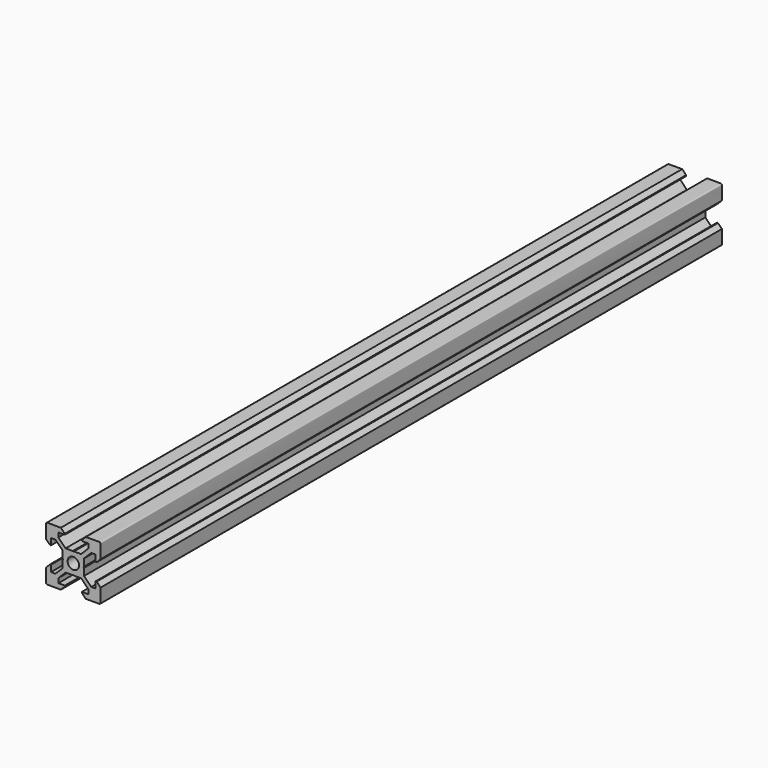
from build123d import *

# Parameters (mm, degrees)
F1_DEPTH = 284.8


# Not quite as in the source:
# - the dataset's text gives a spline's control points without its knots; the knots are read off the source's solid


with BuildPart() as f1:
    # F0 (on Front) → F1 (new body)
    with BuildSketch(Plane.XZ):
        with BuildLine():
            add(Edge.make_bspline(
                [(-8.545, 3.1250000004), (-8.43, 3.1250000004), (-8.315, 3.1250000004), (-8.2, 3.1250000004)],
                knots=[0, 0, 0, 0, 1, 1, 1, 1], degree=3))
            add(Edge.make_bspline(
                [(-8.2, 3.1250000004), (-8.2, 3.9166666671), (-8.2, 4.7083333338), (-8.2, 5.5000000004)],
                knots=[0, 0, 0, 0, 1, 1, 1, 1], degree=3))
            add(Edge.make_bspline(
                [(-8.1999999959, 5.5000000044), (-7.6535533893, 5.5000000044), (-7.1071067826, 5.5000000044), (-6.5606601759, 5.5000000044)],
                knots=[0, 0, 0, 0, 1, 1, 1, 1], degree=3))
            add(Edge.make_bspline(
                [(-6.5606601759, 5.5000000044), (-5.6737734493, 4.6131132778), (-4.7868867226, 3.7262265511), (-3.8999999959, 2.8393398244)],
                knots=[0, 0, 0, 0, 1, 1, 1, 1], degree=3))
            add(Edge.make_bspline(
                [(-3.8999999979, 2.8393398226), (-3.8999999979, 1.9628932159), (-3.8999999979, 1.0864466093), (-3.8999999979, 0.2100000026)],
                knots=[0, 0, 0, 0, 1, 1, 1, 1], degree=3))
            add(Edge.make_bspline(
                [(-3.9, 0.2100000008), (-3.83, 0.1400000008), (-3.76, 0.0700000008), (-3.69, 8e-10)],
                knots=[0, 0, 0, 0, 1, 1, 1, 1], degree=3))
            add(Edge.make_bspline(
                [(-3.9, -0.2099999992), (-3.83, -0.1399999992), (-3.76, -0.0699999992), (-3.69, 8e-10)],
                knots=[0, 0, 0, 0, 1, 1, 1, 1], degree=3))
            add(Edge.make_bspline(
                [(-3.8999999991, -2.839339821), (-3.8999999987, -1.9628932143), (-3.8999999984, -1.0864466077), (-3.899999998, -0.210000001)],
                knots=[0, 0, 0, 0, 1, 1, 1, 1], degree=3))
            add(Edge.make_bspline(
                [(-6.5606601782, -5.5000000017), (-5.6737734512, -4.6131132754), (-4.7868867241, -3.7262265491), (-3.8999999971, -2.8393398228)],
                knots=[0, 0, 0, 0, 1, 1, 1, 1], degree=3))
            add(Edge.make_bspline(
                [(-8.1999999982, -5.5000000011), (-7.6535533915, -5.5000000013), (-7.1071067849, -5.5000000015), (-6.5606601782, -5.5000000017)],
                knots=[0, 0, 0, 0, 1, 1, 1, 1], degree=3))
            add(Edge.make_bspline(
                [(-8.2000000012, -3.1249999971), (-8.2000000015, -3.9166666637), (-8.2000000019, -4.7083333304), (-8.2000000022, -5.4999999971)],
                knots=[0, 0, 0, 0, 1, 1, 1, 1], degree=3))
            add(Edge.make_bspline(
                [(-8.5450000012, -3.1249999969), (-8.4300000012, -3.124999997), (-8.3150000012, -3.124999997), (-8.2000000012, -3.1249999971)],
                knots=[0, 0, 0, 0, 1, 1, 1, 1], degree=3))
            add(Edge.make_bspline(
                [(-10.0000000018, -4.5799999963), (-9.5150000016, -4.0949999965), (-9.0300000014, -3.6099999967), (-8.5450000012, -3.1249999969)],
                knots=[0, 0, 0, 0, 1, 1, 1, 1], degree=3))
            add(Edge.make_bspline(
                [(-10.0000000038, -9.4999999963), (-10.0000000032, -7.8599999963), (-10.0000000025, -6.2199999963), (-10.0000000018, -4.5799999963)],
                knots=[0, 0, 0, 0, 1, 1, 1, 1], degree=3))
            add(Edge.make_bspline(
                [(-9.5000000039, -9.9999999965), (-9.5655199967, -9.9999999965), (-9.6293005688, -9.9873132519), (-9.6913417201, -9.9619397628), (-9.7513299005, -9.9374058943), (-9.8054004587, -9.9012771024), (-9.8535533945, -9.853553387), (-9.8995865416, -9.8079305653), (-9.9357153335, -9.7538600072), (-9.9619397702, -9.6913417126), (-9.9873132593, -9.6308520521), (-10.0000000039, -9.56707148), (-10.0000000038, -9.4999999963)],
                knots=[0, 0, 0, 0, 0.25, 0.25, 0.25, 0.5, 0.5, 0.5, 0.75, 0.75, 0.75, 1, 1, 1, 1], degree=3))
            add(Edge.make_bspline(
                [(-4.580000004, -9.9999999986), (-6.220000004, -9.9999999979), (-7.860000004, -9.9999999972), (-9.500000004, -9.9999999965)],
                knots=[0, 0, 0, 0, 1, 1, 1, 1], degree=3))
            Line((-4.580000004, -9.9999999986), (-3.1250000034, -8.5449999991))
            add(Edge.make_bspline(
                [(-3.1250000033, -8.1999999991), (-3.1250000033, -8.3149999991), (-3.1250000034, -8.4299999991), (-3.1250000034, -8.5449999991)],
                knots=[0, 0, 0, 0, 1, 1, 1, 1], degree=3))
            add(Edge.make_bspline(
                [(-5.5000000033, -8.1999999982), (-4.7083333366, -8.1999999985), (-3.91666667, -8.1999999988), (-3.1250000033, -8.1999999991)],
                knots=[0, 0, 0, 0, 1, 1, 1, 1], degree=3))
            add(Edge.make_bspline(
                [(-5.5000000066, -6.5606601742), (-5.5000000069, -7.1071067808), (-5.5000000071, -7.6535533875), (-5.5000000073, -8.1999999942)],
                knots=[0, 0, 0, 0, 1, 1, 1, 1], degree=3))
            add(Edge.make_bspline(
                [(-2.8393398255, -3.8999999953), (-3.7262265526, -4.7868867216), (-4.6131132796, -5.6737734479), (-5.5000000066, -6.5606601742)],
                knots=[0, 0, 0, 0, 1, 1, 1, 1], degree=3))
            add(Edge.make_bspline(
                [(-0.2100000015, -3.9000000003), (-1.0864466082, -3.9), (-1.9628932149, -3.8999999996), (-2.8393398215, -3.8999999993)],
                knots=[0, 0, 0, 0, 1, 1, 1, 1], degree=3))
            add(Edge.make_bspline(
                [(-1.5e-09, -3.6900000004), (-0.0700000015, -3.7600000004), (-0.1400000015, -3.8300000004), (-0.2100000015, -3.9000000003)],
                knots=[0, 0, 0, 0, 1, 1, 1, 1], degree=3))
            add(Edge.make_bspline(
                [(0.2099999985, -3.9000000005), (0.1399999985, -3.8300000005), (0.0699999985, -3.7600000005), (-1.5e-09, -3.6900000004)],
                knots=[0, 0, 0, 0, 1, 1, 1, 1], degree=3))
            add(Edge.make_bspline(
                [(2.8393398185, -3.9000000016), (1.9628932118, -3.9000000012), (1.0864466051, -3.9000000009), (0.2099999985, -3.9000000005)],
                knots=[0, 0, 0, 0, 1, 1, 1, 1], degree=3))
            add(Edge.make_bspline(
                [(5.4999999974, -6.5606601827), (4.6131132711, -5.6737734557), (3.7262265448, -4.7868867286), (2.8393398185, -3.9000000016)],
                knots=[0, 0, 0, 0, 1, 1, 1, 1], degree=3))
            add(Edge.make_bspline(
                [(5.4999999967, -8.2000000027), (5.4999999969, -7.653553396), (5.4999999971, -7.1071067894), (5.4999999974, -6.5606601827)],
                knots=[0, 0, 0, 0, 1, 1, 1, 1], degree=3))
            add(Edge.make_bspline(
                [(3.1249999967, -8.2000000017), (3.9166666634, -8.200000002), (4.70833333, -8.2000000024), (5.4999999967, -8.2000000027)],
                knots=[0, 0, 0, 0, 1, 1, 1, 1], degree=3))
            add(Edge.make_bspline(
                [(3.1249999966, -8.5450000017), (3.1249999966, -8.4300000017), (3.1249999967, -8.3150000017), (3.1249999967, -8.2000000017)],
                knots=[0, 0, 0, 0, 1, 1, 1, 1], degree=3))
            add(Edge.make_bspline(
                [(4.579999996, -10.0000000023), (4.0949999962, -9.5150000021), (3.6099999964, -9.0300000019), (3.1249999966, -8.5450000017)],
                knots=[0, 0, 0, 0, 1, 1, 1, 1], degree=3))
            add(Edge.make_bspline(
                [(9.499999996, -10.0000000043), (7.859999996, -10.0000000037), (6.219999996, -10.000000003), (4.579999996, -10.0000000023)],
                knots=[0, 0, 0, 0, 1, 1, 1, 1], degree=3))
            add(Edge.make_bspline(
                [(9.999999996, -9.5000000043), (9.999999996, -9.5655199971), (9.9873132515, -9.6293005692), (9.9619397623, -9.6913417205), (9.9374058938, -9.7513299009), (9.9012771019, -9.8054004591), (9.8535533866, -9.853553395), (9.8079305649, -9.899586542), (9.7538600068, -9.9357153339), (9.6913417122, -9.9619397706), (9.6308520517, -9.9873132598), (9.5670714797, -10.0000000043), (9.499999996, -10.0000000043)],
                knots=[0, 0, 0, 0, 0.25, 0.25, 0.25, 0.5, 0.5, 0.5, 0.75, 0.75, 0.75, 1, 1, 1, 1], degree=3))
            add(Edge.make_bspline(
                [(9.9999999981, -4.5800000043), (9.9999999974, -6.2200000043), (9.9999999967, -7.8600000043), (9.999999996, -9.5000000043)],
                knots=[0, 0, 0, 0, 1, 1, 1, 1], degree=3))
            add(Edge.make_bspline(
                [(8.5449999987, -3.1250000037), (9.0299999985, -3.6100000039), (9.5149999983, -4.0950000041), (9.9999999981, -4.5800000043)],
                knots=[0, 0, 0, 0, 1, 1, 1, 1], degree=3))
            add(Edge.make_bspline(
                [(8.1999999987, -3.1250000036), (8.3149999987, -3.1250000036), (8.4299999987, -3.1250000037), (8.5449999987, -3.1250000037)],
                knots=[0, 0, 0, 0, 1, 1, 1, 1], degree=3))
            add(Edge.make_bspline(
                [(8.1999999977, -5.5000000036), (8.199999998, -4.7083333369), (8.1999999983, -3.9166666703), (8.1999999987, -3.1250000036)],
                knots=[0, 0, 0, 0, 1, 1, 1, 1], degree=3))
            add(Edge.make_bspline(
                [(6.5606601777, -5.5000000019), (7.1071067843, -5.5000000022), (7.653553391, -5.5000000024), (8.1999999977, -5.5000000026)],
                knots=[0, 0, 0, 0, 1, 1, 1, 1], degree=3))
            add(Edge.make_bspline(
                [(3.8999999988, -2.8393398208), (4.7868867251, -3.7262265479), (5.6737734514, -4.6131132749), (6.5606601777, -5.5000000019)],
                knots=[0, 0, 0, 0, 1, 1, 1, 1], degree=3))
            add(Edge.make_bspline(
                [(3.8999999999, -0.2100000008), (3.8999999995, -1.0864466075), (3.8999999991, -1.9628932142), (3.8999999988, -2.8393398208)],
                knots=[0, 0, 0, 0, 1, 1, 1, 1], degree=3))
            add(Edge.make_bspline(
                [(3.69, -8e-10), (3.76, -0.0700000008), (3.8299999999, -0.1400000008), (3.8999999999, -0.2100000008)],
                knots=[0, 0, 0, 0, 1, 1, 1, 1], degree=3))
            add(Edge.make_bspline(
                [(3.69, -8e-10), (3.76, 0.0699999992), (3.83, 0.1399999992), (3.9, 0.2099999992)],
                knots=[0, 0, 0, 0, 1, 1, 1, 1], degree=3))
            add(Edge.make_bspline(
                [(3.9, 0.2099999992), (3.9, 1.0864466059), (3.9, 1.9628932126), (3.9, 2.8393398192)],
                knots=[0, 0, 0, 0, 1, 1, 1, 1], degree=3))
            add(Edge.make_bspline(
                [(3.9, 2.8393398192), (4.7868867266, 3.7262265459), (5.6737734533, 4.6131132726), (6.5606601799, 5.4999999992)],
                knots=[0, 0, 0, 0, 1, 1, 1, 1], degree=3))
            add(Edge.make_bspline(
                [(6.5606601799, 5.4999999992), (7.1071067866, 5.4999999992), (7.6535533933, 5.4999999992), (8.2, 5.4999999992)],
                knots=[0, 0, 0, 0, 1, 1, 1, 1], degree=3))
            add(Edge.make_bspline(
                [(8.2, 5.5000000002), (8.2, 4.7083333336), (8.2, 3.9166666669), (8.2, 3.1250000002)],
                knots=[0, 0, 0, 0, 1, 1, 1, 1], degree=3))
            add(Edge.make_bspline(
                [(8.2, 3.1250000002), (8.315, 3.1250000002), (8.43, 3.1250000002), (8.545, 3.1250000002)],
                knots=[0, 0, 0, 0, 1, 1, 1, 1], degree=3))
            add(Edge.make_bspline(
                [(8.545, 3.1250000002), (9.03, 3.6100000002), (9.515, 4.0950000002), (10, 4.5800000002)],
                knots=[0, 0, 0, 0, 1, 1, 1, 1], degree=3))
            add(Edge.make_bspline(
                [(10, 4.5800000002), (10, 6.2200000002), (10, 7.8600000002), (10, 9.5000000002)],
                knots=[0, 0, 0, 0, 1, 1, 1, 1], degree=3))
            add(Edge.make_bspline(
                [(10, 9.5000000002), (10, 9.565519993), (9.9873132554, 9.6293005651), (9.9619397663, 9.6913417164), (9.9374058978, 9.7513298969), (9.901277106, 9.805400455), (9.8535533907, 9.8535533909), (9.807930569, 9.899586538), (9.7538600108, 9.9357153299), (9.6913417163, 9.9619397666), (9.6308520558, 9.9873132558), (9.5670714838, 10.0000000004), (9.5, 10.0000000004)],
                knots=[0, 0, 0, 0, 0.25, 0.25, 0.25, 0.5, 0.5, 0.5, 0.75, 0.75, 0.75, 1, 1, 1, 1], degree=3))
            add(Edge.make_bspline(
                [(9.5, 10.0000000004), (7.86, 10.0000000004), (6.22, 10.0000000004), (4.58, 10.0000000004)],
                knots=[0, 0, 0, 0, 1, 1, 1, 1], degree=3))
            add(Edge.make_bspline(
                [(4.58, 10.0000000004), (4.095, 9.5150000004), (3.61, 9.0300000004), (3.125, 8.5450000004)],
                knots=[0, 0, 0, 0, 1, 1, 1, 1], degree=3))
            add(Edge.make_bspline(
                [(3.125, 8.5450000004), (3.125, 8.4300000004), (3.125, 8.3150000004), (3.125, 8.2000000004)],
                knots=[0, 0, 0, 0, 1, 1, 1, 1], degree=3))
            add(Edge.make_bspline(
                [(3.125, 8.2000000004), (3.9166666667, 8.2000000004), (4.7083333334, 8.2000000004), (5.5, 8.2000000004)],
                knots=[0, 0, 0, 0, 1, 1, 1, 1], degree=3))
            add(Edge.make_bspline(
                [(5.5, 8.2000000004), (5.5, 7.6535533938), (5.5, 7.1071067871), (5.5, 6.5606601804)],
                knots=[0, 0, 0, 0, 1, 1, 1, 1], degree=3))
            add(Edge.make_bspline(
                [(5.5, 6.5606601804), (4.6131132734, 5.6737734538), (3.7262265467, 4.7868867271), (2.8393398201, 3.9000000004)],
                knots=[0, 0, 0, 0, 1, 1, 1, 1], degree=3))
            add(Edge.make_bspline(
                [(2.8393398201, 3.9000000004), (1.9628932134, 3.9000000004), (1.0864466067, 3.9000000004), (0.21, 3.9000000004)],
                knots=[0, 0, 0, 0, 1, 1, 1, 1], degree=3))
            add(Edge.make_bspline(
                [(0.21, 3.9000000004), (0.14, 3.8300000004), (0.07, 3.7600000004), (0, 3.6900000004)],
                knots=[0, 0, 0, 0, 1, 1, 1, 1], degree=3))
            add(Edge.make_bspline(
                [(0, 3.6900000004), (-0.07, 3.7600000004), (-0.14, 3.8300000004), (-0.21, 3.9000000004)],
                knots=[0, 0, 0, 0, 1, 1, 1, 1], degree=3))
            add(Edge.make_bspline(
                [(-0.21, 3.9000000004), (-1.0864466066, 3.9000000004), (-1.9628932133, 3.9000000004), (-2.8393398199, 3.9000000004)],
                knots=[0, 0, 0, 0, 1, 1, 1, 1], degree=3))
            add(Edge.make_bspline(
                [(-2.8393398239, 3.8999999964), (-3.7262265506, 4.7868867231), (-4.6131132773, 5.6737734498), (-5.5000000039, 6.5606601764)],
                knots=[0, 0, 0, 0, 1, 1, 1, 1], degree=3))
            add(Edge.make_bspline(
                [(-5.5, 6.5606601804), (-5.5, 7.1071067871), (-5.5, 7.6535533938), (-5.5, 8.2000000004)],
                knots=[0, 0, 0, 0, 1, 1, 1, 1], degree=3))
            add(Edge.make_bspline(
                [(-5.5, 8.2000000004), (-4.7083333333, 8.2000000004), (-3.9166666666, 8.2000000004), (-3.125, 8.2000000004)],
                knots=[0, 0, 0, 0, 1, 1, 1, 1], degree=3))
            add(Edge.make_bspline(
                [(-3.125, 8.2000000004), (-3.125, 8.3150000004), (-3.125, 8.4300000004), (-3.125, 8.5450000004)],
                knots=[0, 0, 0, 0, 1, 1, 1, 1], degree=3))
            Line((-3.125, 8.5450000004), (-4.58, 10.0000000004))
            add(Edge.make_bspline(
                [(-4.58, 10.0000000004), (-6.22, 10.0000000004), (-7.86, 10.0000000004), (-9.5, 10.0000000004)],
                knots=[0, 0, 0, 0, 1, 1, 1, 1], degree=3))
            add(Edge.make_bspline(
                [(-9.4999999998, 10.0000000004), (-9.5655199926, 10.0000000005), (-9.6293005647, 9.9873132559), (-9.691341716, 9.9619397667), (-9.7513298965, 9.9374058983), (-9.8054004546, 9.9012771064), (-9.8535533905, 9.8535533911), (-9.8995865376, 9.8079305694), (-9.9357153295, 9.7538600112), (-9.9619397662, 9.6913417167), (-9.9873132554, 9.6308520562), (-10, 9.5670714842), (-10, 9.5000000004)],
                knots=[0, 0, 0, 0, 0.25, 0.25, 0.25, 0.5, 0.5, 0.5, 0.75, 0.75, 0.75, 1, 1, 1, 1], degree=3))
            add(Edge.make_bspline(
                [(-10, 9.5000000004), (-10, 7.8600000004), (-10, 6.2200000004), (-10, 4.5800000004)],
                knots=[0, 0, 0, 0, 1, 1, 1, 1], degree=3))
            add(Edge.make_bspline(
                [(-10, 4.5800000004), (-9.515, 4.0950000004), (-9.03, 3.6100000004), (-8.545, 3.1250000004)],
                knots=[0, 0, 0, 0, 1, 1, 1, 1], degree=3))
        make_face()
        with BuildLine():
            add(Edge.make_bspline(
                [(2.1, -4e-10), (2.1000000002, 0.2748893568), (1.9906569307, 0.8245399239), (1.5235828541, 1.5235874774), (0.8245570992, 1.9906556095), (5e-10, 2.1546721958), (-0.8245570982, 1.9906556098), (-1.5235828533, 1.523587478), (-1.9906569302, 0.8245399247), (-2.1, 0.2748893577), (-2.1, 4e-10)],
                knots=[-3.1415926536, -3.1415926536, -3.1415926536, -3.1415926536, -2.7488935719, -2.3561944902, -1.9634954085, -1.5707963268, -1.1780972451, -0.7853981634, -0.3926990817, 0, 0, 0, 0], degree=3))
            add(Edge.make_bspline(
                [(2.1, -4e-10), (2.1, -0.2748893577), (1.9906569304, -0.8245399247), (1.5235828534, -1.523587478), (0.8245570983, -1.9906556098), (-4e-10, -2.1546721958), (-0.824557099, -1.9906556095), (-1.5235828539, -1.5235874774), (-1.9906569306, -0.8245399239), (-2.1, -0.2748893568), (-2.1, 4e-10)],
                knots=[-3.1415926536, -3.1415926536, -3.1415926536, -3.1415926536, -2.7488935719, -2.3561944902, -1.9634954085, -1.5707963268, -1.1780972451, -0.7853981634, -0.3926990817, 0, 0, 0, 0], degree=3))
        make_face(mode=Mode.SUBTRACT)
    extrude(amount=-F1_DEPTH)


solid = f1.part
